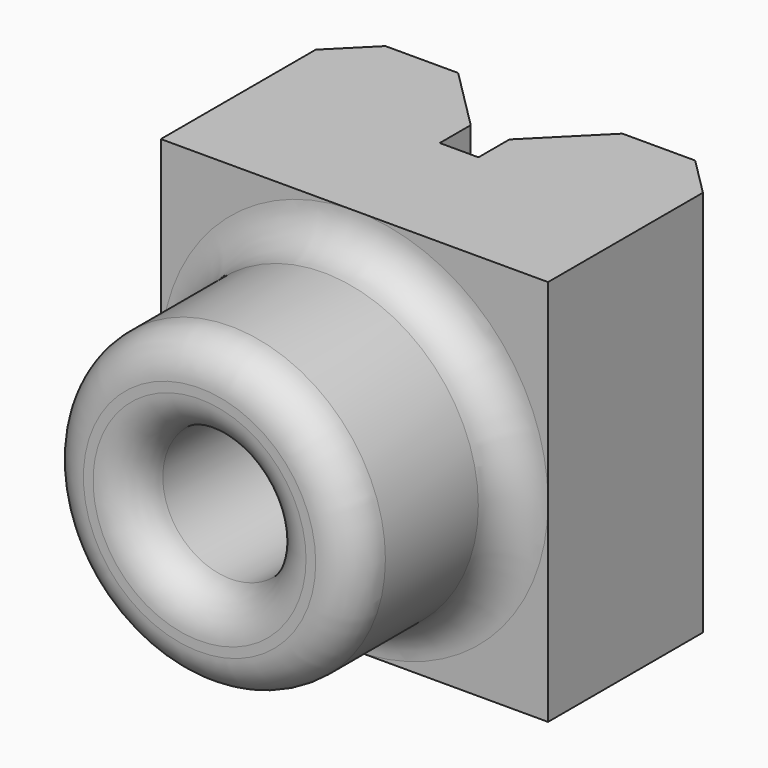
from build123d import *

# Parameters (mm, degrees)
F1_DEPTH = 10
F2_R     = 4
F2_R_2   = 1.75
F3_DEPTH = 5
F4_SIZE  = 1
F5_W     = 1
F5_H     = 2.3880545414
F6_DEPTH = 25
F7_R     = 0.99999


# Not quite as in the source:
# - a fillet or chamfer is up to 0.001 mm smaller than in the source, because OpenCascade refuses the exact size


with BuildPart() as f1:
    # F0 (on Top) → F1 (new body)
    with BuildSketch(Plane.XY):
        Polygon((0, 6), (0, 0), (10, 0), (10, 6), (7.1213203436, 6), (5, 3.8786796564), (2.8786796564, 6), align=None)
    extrude(amount=F1_DEPTH)

    # F2 (on face) → F3 (join)
    with BuildSketch(Plane.XZ):
        with Locations((5, 5)):
            Circle(F2_R)
        with Locations((5, 5)):
            Circle(F2_R_2, mode=Mode.SUBTRACT)
    extrude(amount=F3_DEPTH)

    # F4
    f4_edges = [f1.edges().sort_by_distance(p)[0] for p in [
        (10, 6, 5),
        (0, 6, 5),
    ]]
    chamfer(f4_edges, length=F4_SIZE)

    # F5 (on face) → F6 (cut)
    with BuildSketch(Plane(origin=(0, 0, 0), x_dir=(1, 0, 0), z_dir=(0, 0, -1))):
        with Locations((5, -4.5727069271)):
            Rectangle(F5_W, F5_H)
    extrude(amount=-F6_DEPTH, mode=Mode.SUBTRACT)

    # F7 (radius 1 in the source; OpenCascade refuses exactly that, so slightly less here)
    f7_edges = [f1.edges().sort_by_distance(p)[0] for p in [
        (1, 0, 5),
        (1, -5, 5),
        (3.25, -5, 5),
    ]]
    fillet(f7_edges, radius=F7_R)


solid = f1.part
